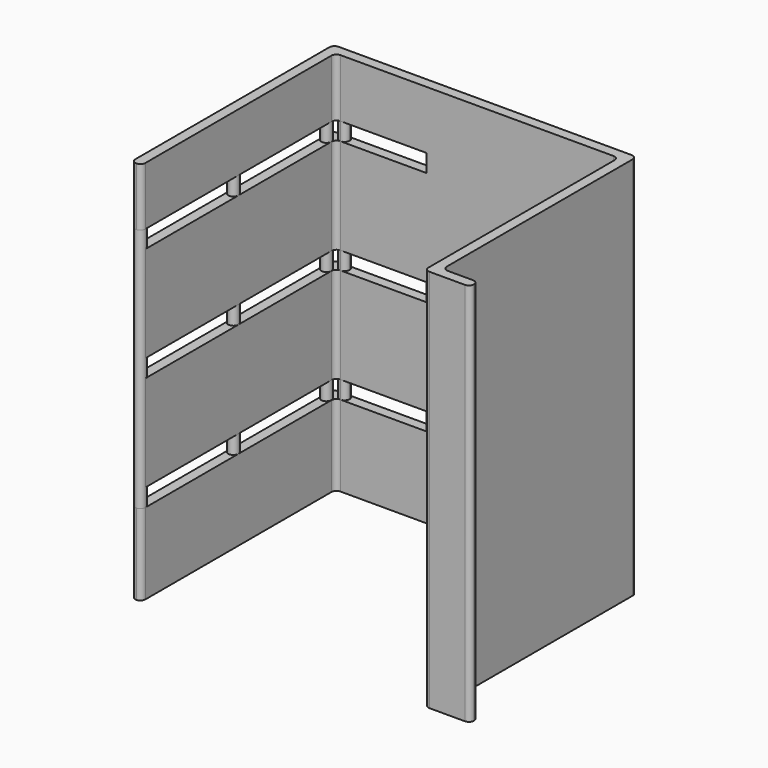
from build123d import *

# Parameters (mm, degrees)
F1_DEPTH = 76
F2_W     = 1
F2_H     = 3.5
F2_W_2   = 19
F3_DEPTH = 50.001
F5_DEPTH = 48.5


# Not quite as in the source:
# - a feature names something its author has since deleted; it is built from what else it names


with BuildPart() as f1:
    # F0 (on Top) → F1 (new body)
    with BuildSketch(Plane.XY):
        with BuildLine():
            ThreePointArc((-1, 0), (-0.2928932188, 0.2928932188), (0, 1))
            Line((0, 1), (0, 47))
            ThreePointArc((0, 47), (0.2928932188, 47.7071067812), (1, 48))
            Line((1, 48), (55, 48))
            ThreePointArc((55, 48), (55.7071067812, 47.7071067812), (56, 47))
            Line((56, 47), (56, 1))
            ThreePointArc((56, 1), (56.2928932188, 0.2928932188), (57, 0))
            Line((57, 0), (64, 0))
            ThreePointArc((64, 0), (64.7071067812, 0.2928932188), (65, 1))
            ThreePointArc((65, 1), (64.7071067812, 1.7071067812), (64, 2))
            Line((64, 2), (59, 2))
            ThreePointArc((59, 2), (58.2928932188, 2.2928932188), (58, 3))
            Line((58, 3), (58, 49))
            ThreePointArc((58, 49), (57.7071067812, 49.7071067812), (57, 50))
            Line((57, 50), (-1, 50))
            ThreePointArc((-1, 50), (-1.7071067812, 49.7071067812), (-2, 49))
            Line((-2, 49), (-2, 1))
            ThreePointArc((-2, 1), (-1.7071067812, 0.2928932188), (-1, 0))
        make_face()
    extrude(amount=F1_DEPTH)

    # F2 (on face) → F3 (cut, through all)
    with BuildSketch(Plane(origin=(0, 50, 0), x_dir=(-1, 0, 0), z_dir=(0, 1, 0))):
        with Locations((1.5, 17.75)):
            Rectangle(F2_W, F2_H)
        with Locations((-8.5, 17.75)):
            Rectangle(F2_W_2, F2_H)
        with Locations((-8.5, 40.25)):
            Rectangle(F2_W_2, F2_H)
        with Locations((-8.5, 62.75)):
            Rectangle(F2_W_2, F2_H)
        with Locations((1.5, 40.25)):
            Rectangle(F2_W, F2_H)
        with Locations((1.5, 62.75)):
            Rectangle(F2_W, F2_H)
    extrude(amount=-F3_DEPTH, mode=Mode.SUBTRACT)

    # F4 (on face) → F5 (join, through all)
    with BuildSketch(Plane.XY.offset(16)):
        with BuildLine():
            ThreePointArc((0, 47), (-1, 48), (-2, 47))
            ThreePointArc((-2, 47), (-1, 46), (0, 47))
        make_face()
        with BuildLine():
            ThreePointArc((0, 24), (-1, 25), (-2, 24))
            ThreePointArc((-2, 24), (-1, 23), (0, 24))
        make_face()
        with BuildLine():
            ThreePointArc((0, 1), (-1, 2), (-2, 1))
            ThreePointArc((-2, 1), (-1, 0), (0, 1))
        make_face()
        with BuildLine():
            ThreePointArc((0.999999997, 50), (0, 48.9999999985), (1, 48))
            ThreePointArc((1, 48), (1.7071067812, 48.2928932188), (2, 49))
            ThreePointArc((2, 49), (1.7071067801, 49.7071067822), (0.999999997, 50))
        make_face()
    extrude(amount=F5_DEPTH)


solid = f1.part
